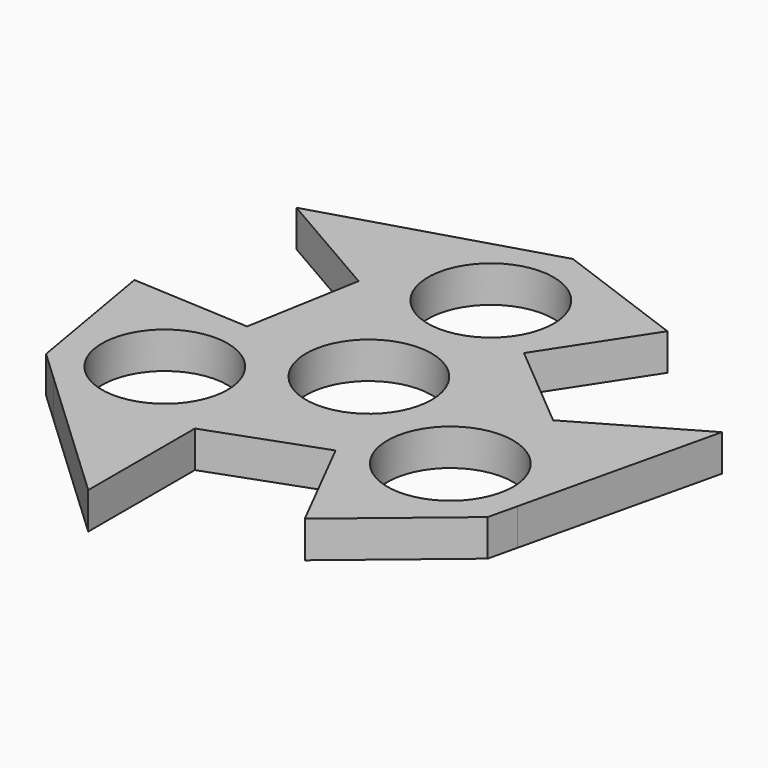
from build123d import *

# Parameters (mm, degrees)
F0_R     = 10.9
F1_DEPTH = 6.35


# Not quite as in the source:
# - a length typed as a fraction of an inch, garbled in the dataset ("3 / 203.2 mm" for 3/8 in), is restored


with BuildPart() as f1:
    # F0 (on Top) → F1 (new body)
    with BuildSketch(Plane.XY):
        Polygon((12.0834760459, 18.5353325598), (23.2533272356, 35.6692190058), (0, 44.2333527703), (-8.7317753371, 41.5979945749), (-38.6247036873, 32.5759376999), (-18.593203622, 21.0107457448), (-22.0938068874, 1.1969309419), (-42.51711341, 2.3033626056), (-38.3072071936, -22.1166763852), (-34.5838293668, -25.6138377102), (-32.9914432749, -27.1094772381), (-8.8992377565, -49.7379434568), (-8.8992377565, -26.6075595468), (10.0103308414, -19.7322635017), (19.2637861744, -37.9725816114), (38.3072071936, -22.1166763852), (39.4741488289, -17.1435559367), (39.973217609, -15.0166893646), (47.5239414439, 17.162005757), (27.4924413785, 5.5968138019), align=None)
        with Locations((-23.4244655113, -14.9711193807)):
            Circle(F0_R, mode=Mode.SUBTRACT)
        with Locations((24.5570029423, -13.0304875769)):
            Circle(F0_R, mode=Mode.SUBTRACT)
        Circle(F0_R, mode=Mode.SUBTRACT)
        with Locations((-1.0652008007, 27.7795850807)):
            Circle(F0_R, mode=Mode.SUBTRACT)
    extrude(amount=F1_DEPTH)


solid = f1.part
